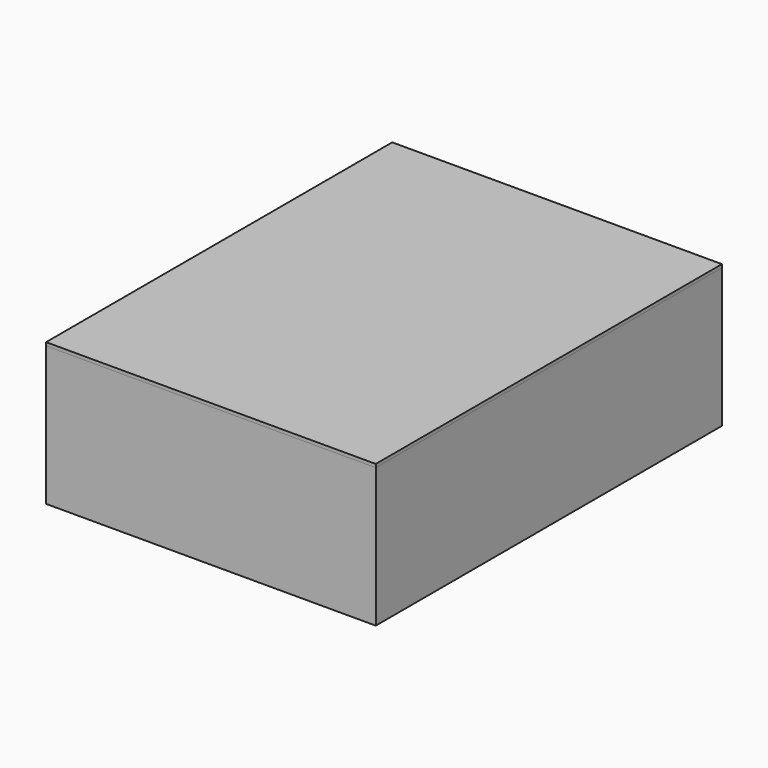
from build123d import *

# Parameters (mm, degrees)
F0_W     = 25.4
F0_H     = 10.715625
F1_DEPTH = 33.3375
F2_W     = 25.4
F2_H     = 0.254
F3_DEPTH = 33.3375


# Not quite as in the source:
# - a feature names something its author has since deleted; it is built from what else it names


with BuildPart() as f1:
    # F0 (on Front) → F1 (new body)
    with BuildSketch(Plane.XZ):
        with Locations((12.7, 5.3578125)):
            Rectangle(F0_W, F0_H)
    extrude(amount=F1_DEPTH)


with BuildPart() as f3:
    # F2 (on Front) → F3 (new body)
    with BuildSketch(Plane.XZ):
        with Locations((12.7, 10.842625)):
            Rectangle(F2_W, F2_H)
    extrude(amount=F3_DEPTH)


solid = Compound([f1.part, f3.part])
